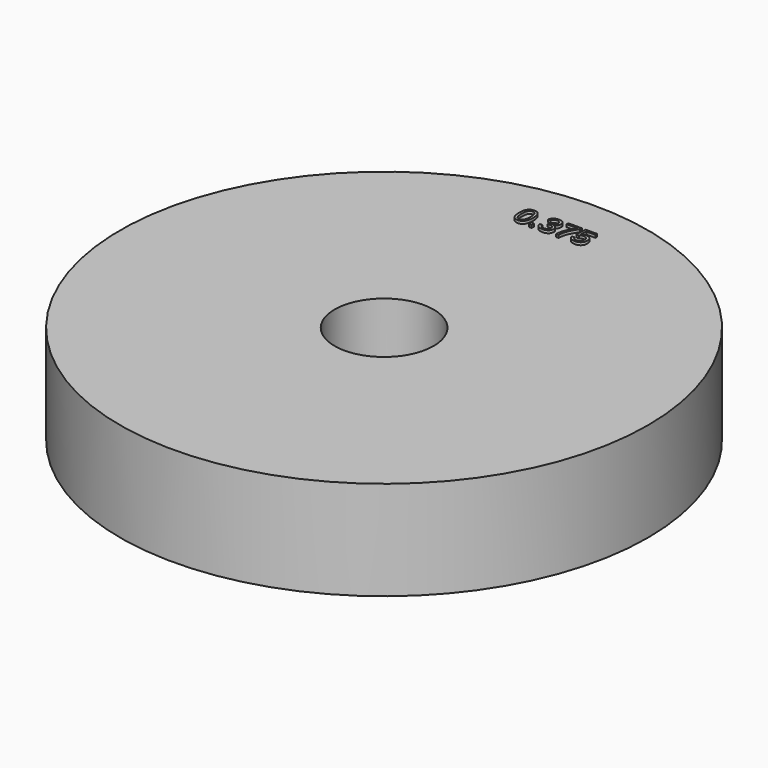
from build123d import *

# Parameters (mm, degrees)
F0_R         = 25.4
F0_R_2       = 4.7625
F1_DEPTH     = 9.525
F2_TEXT_SIZE = 2.8292784912
F3_DEPTH     = 0.254


# Not quite as in the source:
# - Text() gives the source's letters only with a copy of the font that has no kerning and outlines rounded to 1/6400 em; it was checked with that copy


with BuildPart() as f1:
    # F0 (on Top) → F1 (new body)
    with BuildSketch(Plane.XY):
        Circle(F0_R)
        Circle(F0_R_2, mode=Mode.SUBTRACT)
    extrude(amount=F1_DEPTH)

    # F2 (on face) → F3 (join)
    with BuildSketch(Plane.XY.offset(9.525)):
        with Locations((-3.5785952166, 19.600937143)):
            Text('0.375', F2_TEXT_SIZE, font='Arimo', text_align=(TextAlign.LEFT, TextAlign.BOTTOM))
    extrude(amount=F3_DEPTH)


solid = f1.part
